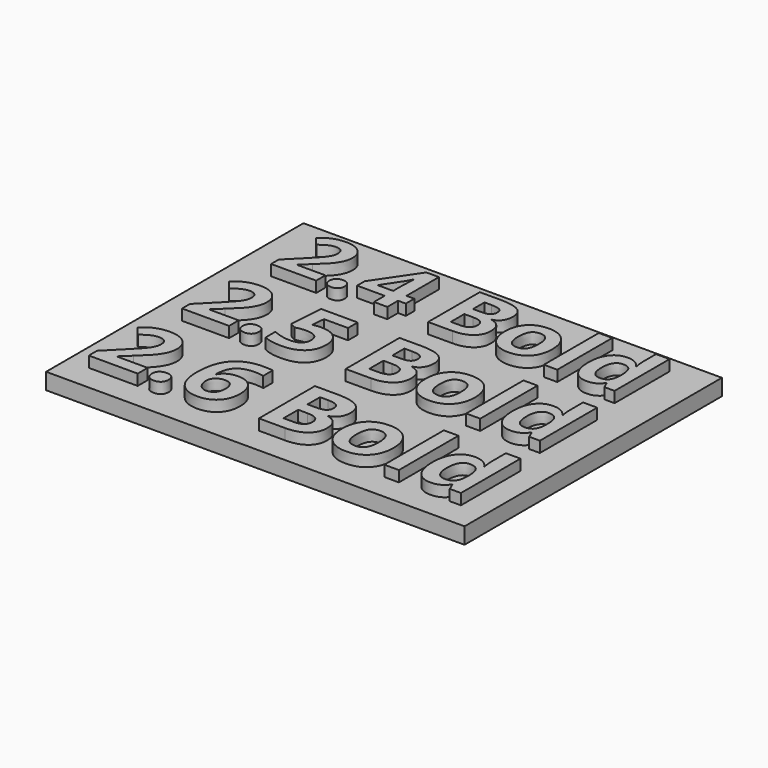
from build123d import *

# Parameters (mm, degrees)
F0_TEXT_SIZE   = 3.3333333333
F0_TEXT_SIZE_2 = 3.4722222222
F0_TEXT_SIZE_3 = 3.6111111111
F2_DEPTH       = 1
F1_W           = 15.4210836627
F1_H           = 11.8574122898
F3_DEPTH       = 0.6


# Not quite as in the source:
# - Text() gives the source's letters only with a copy of the font that has no kerning and outlines rounded to 1/6400 em; it was checked with that copy


with BuildPart() as f2:
    # F0 (on Top) → F2 (new body)
    with BuildSketch(Plane.XY):
        with Locations((-23.3441257661, 16.6067173579)):
            Text('2.4 Bold', F0_TEXT_SIZE, font='Open Sans', font_style=FontStyle.BOLD, text_align=(TextAlign.LEFT, TextAlign.BOTTOM))
        with Locations((-23.615154412, 12.8388810346)):
            Text('2.5 Bold', F0_TEXT_SIZE_2, font='Open Sans', font_style=FontStyle.BOLD, text_align=(TextAlign.LEFT, TextAlign.BOTTOM))
        with Locations((-23.8861830578, 8.8734701656)):
            Text('2.6 Bold', F0_TEXT_SIZE_3, font='Open Sans', font_style=FontStyle.BOLD, text_align=(TextAlign.LEFT, TextAlign.BOTTOM))
    extrude(amount=F2_DEPTH)

    # F1 (on Top) → F3 (join)
    with BuildSketch(Plane.XY):
        with Locations((-16.8394382661, 13.8451985844)):
            Rectangle(F1_W, F1_H)
    extrude(amount=F3_DEPTH)


solid = f2.part
